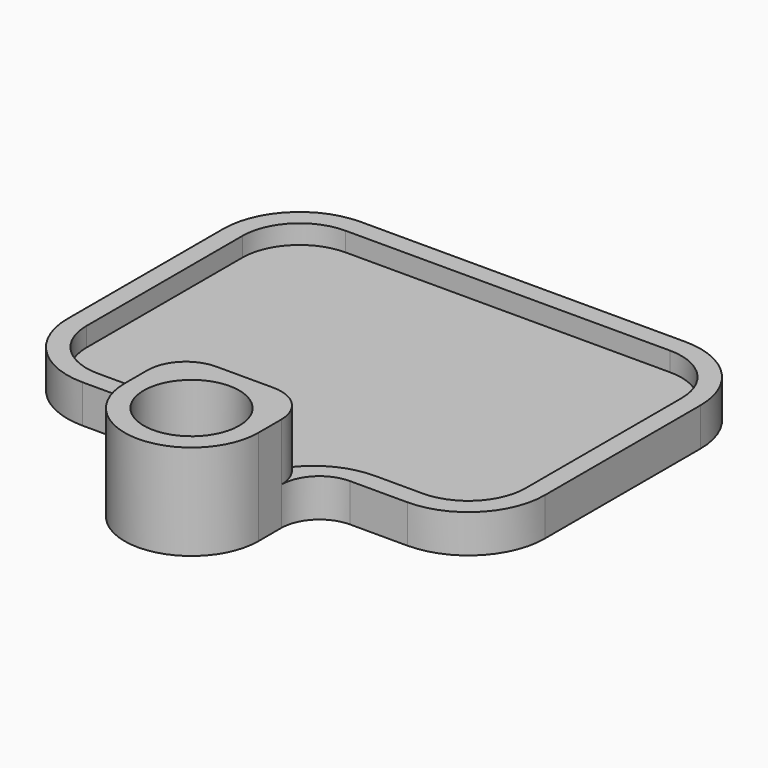
from build123d import *

# Parameters (mm, degrees)
F0_R         = 12.5
F1_DEPTH     = 10
F2_R         = 12.5
F3_DEPTH     = 15
F4_T         = 5
F4_T3_DEPTH  = 20
F5_R         = 10
F6_T1_DEPTH  = 40
F7_T1_DEPTH  = 5
F7_T6_DEPTH  = 92.3194198861
F7_T13_DEPTH = 48.659709943


# Not quite as in the source:
# - a fillet or chamfer that OpenCascade refuses, or shapes differently, is made with other operations: its cross-section is extruded or revolved along the edge and cut away or added
# - a shell that OpenCascade refuses in one call is made with other operations: the cavity is built on its own and cut out


with BuildPart() as f1:
    # F0 (on Top) → F1 (new body)
    with BuildSketch(Plane.XY):
        with BuildLine():
            Line((17.5, 0), (17.5, 17.5))
            Line((17.5, 17.5), (0, 17.5))
            ThreePointArc((0, 17.5), (12.3743686708, 12.3743686708), (17.5, 0))
        make_face()
        with BuildLine():
            Line((0, 17.5), (-17.5, 17.5))
            Line((-17.5, 17.5), (-17.5, 0))
            ThreePointArc((-17.5, 0), (-12.3743686708, 12.3743686708), (0, 17.5))
        make_face()
        with BuildLine():
            ThreePointArc((17.5, 0), (12.3743686708, 12.3743686708), (0, 17.5))
            ThreePointArc((0, 17.5), (-12.3743686708, 12.3743686708), (-17.5, 0))
            ThreePointArc((-17.5, 0), (0, -17.5), (17.5, 0))
        make_face()
        Circle(F0_R, mode=Mode.SUBTRACT)
        with BuildLine():
            Line((42.5, 108.5), (0, 108.5))
            Line((0, 108.5), (-42.5, 108.5))
            ThreePointArc((-42.5, 108.5), (-56.6421356237, 102.6421356237), (-62.5, 88.5))
            Line((-62.5, 88.5), (-62.5, 37.5))
            ThreePointArc((-62.5, 37.5), (-56.6421356237, 23.3578643763), (-42.5, 17.5))
            Line((-42.5, 17.5), (-17.5, 17.5))
            Line((-17.5, 17.5), (0, 17.5))
            Line((0, 17.5), (17.5, 17.5))
            Line((17.5, 17.5), (42.5, 17.5))
            ThreePointArc((42.5, 17.5), (56.6421356237, 23.3578643763), (62.5, 37.5))
            Line((62.5, 37.5), (62.5, 88.5))
            ThreePointArc((62.5, 88.5), (56.6421356237, 102.6421356237), (42.5, 108.5))
        make_face()
    extrude(amount=F1_DEPTH)

    # F2 (on face) → F3 (join)
    with BuildSketch(Plane.XY.offset(10)):
        with BuildLine():
            Line((17.5, 17.5), (-17.5, 17.5))
            Line((-17.5, 17.5), (-17.5, 0))
            ThreePointArc((-17.5, 0), (0, -17.5), (17.5, 0))
            Line((17.5, 0), (17.5, 17.5))
        make_face()
        Circle(F2_R, mode=Mode.SUBTRACT)
    extrude(amount=F3_DEPTH)

    # F4: shell of thickness 5, made by hand


with BuildPart() as f4_core1:
    # F4_t2: copy of F1
    add(f1.part)

    # the walls: a layer under each face that stays
    f4_faces = [f4_core1.faces().sort_by_distance(p)[0] for p in [
        (0, -17.5, 12.5),
        (0, 45.5, 0),
        (-12.5, 0, 12.5),
        (-30, 17.5, 5),
        (0, 17.5, 17.5),
        (-56.6421356237, 23.3578643763, 5),
        (-62.5, 63, 5),
        (-56.6421356237, 102.6421356237, 5),
        (0, 108.5, 5),
        (56.6421356237, 102.6421356237, 5),
        (62.5, 63, 5),
        (56.6421356237, 23.3578643763, 5),
        (30, 17.5, 5),
        (17.5, 8.75, 12.5),
        (-11.6666666667, -11.6666666667, 25),
        (-17.5, 8.75, 12.5),
    ]]
    thicken(f4_faces, amount=-F4_T, mode=Mode.SUBTRACT)

    # F4_s4 → F4_t3 (cut)
    with BuildSketch(Plane.XY.offset(-5)):
        Polygon((-17.55, 17.45), (-17.5, 22.5), (-12.5, 22.5), (-12.5, 17.5), align=None)
        Polygon((17.55, 17.45), (17.5, 22.5), (12.5, 22.5), (12.5, 17.5), align=None)
    extrude(amount=F4_T3_DEPTH, mode=Mode.SUBTRACT)


with BuildPart() as f1_1:
    add(f1.part)

    # what is left inside the walls is the cavity
    f4_cavity = [f4_core1.part.solids().sort_by_distance(p)[0] for p in [
        (0, 42.664966, 5.05),
    ]]
    add(f4_cavity, mode=Mode.SUBTRACT)

    # F5
    f5_edges = [f1_1.edges().sort_by_distance(p)[0] for p in [
        (17.5, 17.5, 5),
        (-17.5, 17.5, 5),
    ]]
    fillet(f5_edges, radius=F5_R)

    # F6: fillet of radius 10 on 2 edges, made by hand

    # F6_s2 → F6_t1 (cut)
    with BuildSketch(Plane.XY.offset(10)):
        with BuildLine():
            ThreePointArc((7.5, 17.5), (14.5710678119, 14.5710678119), (17.5, 7.5))
            Line((17.5, 7.5), (17.5, 17.5))
            Line((17.5, 17.5), (7.5, 17.5))
        make_face()
        with BuildLine():
            ThreePointArc((-17.5, 7.5), (-14.5710678119, 14.5710678119), (-7.5, 17.5))
            Line((-7.5, 17.5), (-17.5, 17.5))
            Line((-17.5, 17.5), (-17.5, 7.5))
        make_face()
    extrude(amount=F6_T1_DEPTH, mode=Mode.SUBTRACT)

    # F7: fillet of radius 20 on 2 edges, made by hand

    # F7_s2 → F7_t1 (cut)
    with BuildSketch(Plane.XY.offset(5)):
        with BuildLine():
            ThreePointArc((12.5, 12.2474487139), (19.8383956996, 19.7474487139), (29.9638839772, 22.5))
            Line((29.9638839772, 22.5), (12.5, 22.5))
            Line((12.5, 22.5), (12.5, 12.2474487139))
        make_face()
        with BuildLine():
            ThreePointArc((-29.9638839772, 22.5), (-19.8383956996, 19.7474487139), (-12.5, 12.2474487139))
            Line((-12.5, 12.2474487139), (-12.5, 22.5))
            Line((-12.5, 22.5), (-29.9638839772, 22.5))
        make_face()
    extrude(amount=F7_T1_DEPTH, mode=Mode.SUBTRACT)


with BuildPart() as f7_tool4:
    # F7_s5 → F7_t6 (new body)
    with BuildSketch(Plane.XY.offset(-38.659709943)):
        with BuildLine():
            ThreePointArc((12.5, 12.2474487139), (19.8383956996, 19.7474487139), (29.9638839772, 22.5))
            Line((29.9638839772, 22.5), (12.5, 22.5))
            Line((12.5, 22.5), (12.5, 12.2474487139))
        make_face()
    extrude(amount=F7_T6_DEPTH)

    split(bisect_by=Plane.XZ.offset(-12.5), keep=Keep.TOP)

    split(bisect_by=Plane.XY.offset(20), keep=Keep.BOTTOM)

    split(bisect_by=Plane.XY.offset(10), keep=Keep.TOP)


with BuildPart() as f1_2:
    add(f1_1.part)

    # F7_t3: cut F7_tool4
    add(f7_tool4.part, mode=Mode.SUBTRACT)


with BuildPart() as f7_tool11:
    # F7_s12 → F7_t13 (new body)
    with BuildSketch(Plane.XY.offset(5)):
        with BuildLine():
            ThreePointArc((-29.9638839772, 22.5), (-19.8383956996, 19.7474487139), (-12.5, 12.2474487139))
            Line((-12.5, 12.2474487139), (-12.5, 22.5))
            Line((-12.5, 22.5), (-29.9638839772, 22.5))
        make_face()
    extrude(amount=F7_T13_DEPTH)

    split(bisect_by=Plane.XZ.offset(-12.5), keep=Keep.TOP)

    split(bisect_by=Plane.XY.offset(20), keep=Keep.BOTTOM)


with BuildPart() as f1_3:
    add(f1_2.part)

    # F7_t10: cut F7_tool11
    add(f7_tool11.part, mode=Mode.SUBTRACT)


solid = f1_3.part
